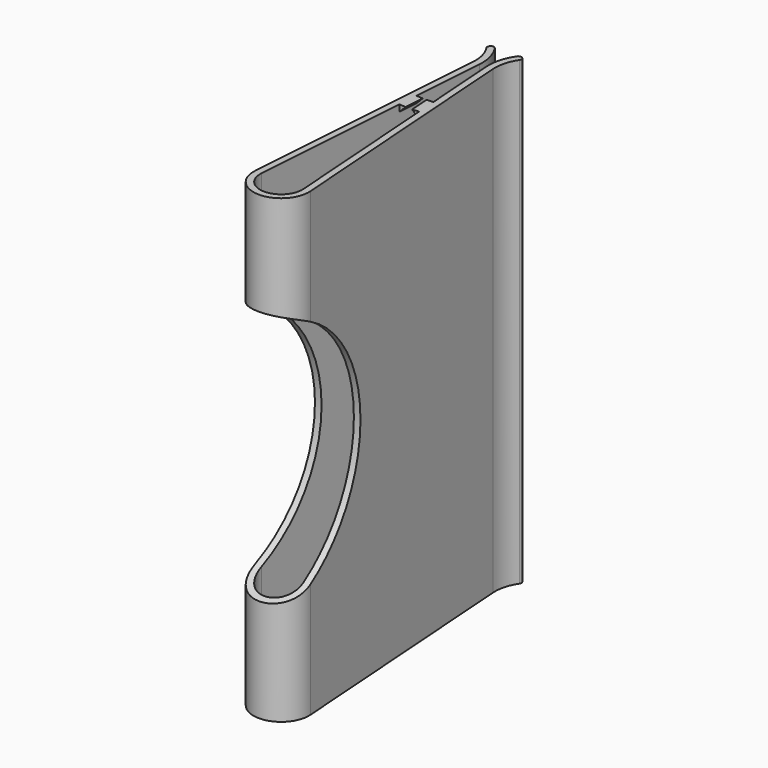
from build123d import *

# Parameters (mm, degrees)
F1_DEPTH = 88.9
F3_DEPTH = 1.27
F5_DEPTH = 1.27
F6_SIZE  = 1.26999
F8_DEPTH = 12.7


# Not quite as in the source:
# - a fillet or chamfer is up to 0.001 mm smaller than in the source, because OpenCascade refuses the exact size


with BuildPart() as f1:
    # F0 (on Top) → F1 (new body)
    with BuildSketch(Plane.XY):
        with BuildLine():
            Line((-4.064, 0), (-0.635, 48.26))
            ThreePointArc((-0.635, 48.26), (-0.9122099758, 51.1784184141), (-2.1235503767, 53.848))
            ThreePointArc((-2.1235503767, 53.848), (-3.0047663986, 54.0209402292), (-3.1777066278, 53.1397242074))
            ThreePointArc((-3.1777066278, 53.1397242074), (-2.1394148555, 50.8515114195), (-1.9018063048, 48.3500099217))
            Line((-1.9018063048, 48.3500099217), (-5.3308063048, 0.0900099217))
            ThreePointArc((-5.3308063048, 0.0900099217), (0, -5.633003484), (5.3308063048, 0.0900099217))
            Line((5.3308063048, 0.0900099217), (1.9018063048, 48.3500099217))
            ThreePointArc((1.9018063048, 48.3500099217), (2.1394148555, 50.8515114195), (3.1777066278, 53.1397242074))
            ThreePointArc((3.1777066278, 53.1397242074), (3.0047663986, 54.0209402292), (2.1235503767, 53.848))
            ThreePointArc((2.1235503767, 53.848), (0.9122099758, 51.1784184141), (0.635, 48.26))
            Line((0.635, 48.26), (4.064, 0))
            ThreePointArc((4.064, 0), (0, -4.363003484), (-4.064, 0))
        make_face()
    extrude(amount=F1_DEPTH)

    # F2 (on face) → F3 (join)
    with BuildSketch(Plane.XY.offset(88.9)):
        Polygon((-0.3550842778, 34.2804189145), (-1.6218905827, 34.3704288362), (-1.8919203477, 30.5700099217), (-0.6251140428, 30.48), align=None)
        Polygon((0.6251140428, 30.48), (1.8919203477, 30.5700099217), (1.6218905827, 34.3704288362), (0.3550842778, 34.2804189145), align=None)
    extrude(amount=-F3_DEPTH)

    # F4 (on face) → F5 (join)
    with BuildSketch(Plane(origin=(0, 0, 0), x_dir=(1, 0, 0), z_dir=(0, 0, -1))):
        Polygon((-0.6251140428, -30.48), (-1.8919203477, -30.5700099217), (-1.6218905827, -34.3704288362), (-0.3550842778, -34.2804189145), align=None)
        Polygon((1.6218905827, -34.3704288362), (1.8919203477, -30.5700099217), (0.6251140428, -30.48), (0.3550842778, -34.2804189145), align=None)
    extrude(amount=-F5_DEPTH)

    # F6 (size 1.27 in the source; OpenCascade refuses exactly that, so slightly less here)
    f6_edges = [f1.edges().sort_by_distance(p)[0] for p in [
        (-0.490099, 32.380209, 1.27),
        (0.490099, 32.380209, 1.27),
        (-0.490099, 32.380209, 87.63),
        (0.490099, 32.380209, 87.63),
    ]]
    chamfer(f6_edges, length=F6_SIZE)

    # F7 (on Right) → F8 (cut, symmetric)
    with BuildSketch(Plane.YZ):
        with BuildLine():
            ThreePointArc((-5.842, 19.8251978841), (13.3307116053, 44.45), (-5.842, 69.0748021159))
            Line((-5.842, 69.0748021159), (-5.842, 19.8251978841))
        make_face()
    extrude(amount=F8_DEPTH, both=True, mode=Mode.SUBTRACT)


solid = f1.part
